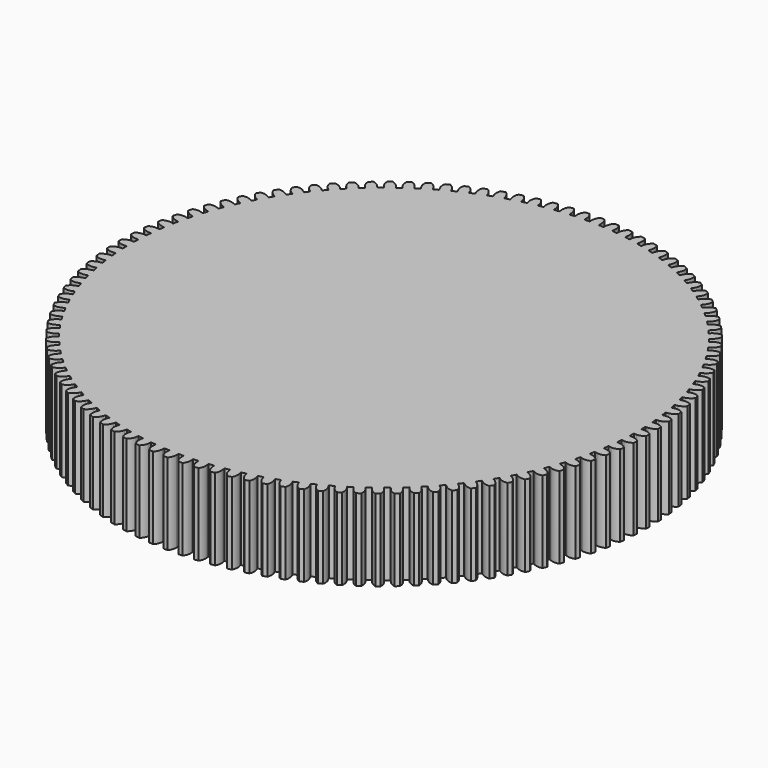
from build123d import *

# Parameters (mm, degrees)
F0_R            = 82.1730673952
F1_DEPTH        = 25.4
F3_DEPTH        = 25.4
F3_COPIES_COUNT = 110


# Not quite as in the source:
# - a pattern or mirror of a feature is missing from the dataset's text; its kind, count and spacing are read off the source's solid


with BuildPart() as f1:
    # F0 (on Top) → F1 (new body)
    with BuildSketch(Plane.XY):
        Circle(F0_R)
    extrude(amount=F1_DEPTH)

    # F2 (on face) → F3 (cut, through all)
    with BuildSketch(Plane.XY.offset(25.4)):
        with BuildLine():
            Line((-0.79375, 79.7918173952), (-0.79375, 78.9980673952))
            Line((-0.79375, 78.9980673952), (0.79375, 78.9980673952))
            Line((0.79375, 78.9980673952), (0.79375, 79.7918173952))
            ThreePointArc((0.79375, 79.7918173952), (1.0268322874, 81.0567714657), (1.6954639006, 82.155574414))
            ThreePointArc((1.6954639006, 82.155574414), (0, 82.1730673952), (-1.6954639006, 82.155574414))
            ThreePointArc((-1.6954639006, 82.155574414), (-1.0268322874, 81.0567714657), (-0.79375, 79.7918173952))
        make_face()
    f3 = extrude(amount=-F3_DEPTH, mode=Mode.SUBTRACT)

    # F3_copies: F3 ×110 about axis
    f3_copies_axis = Axis((0, 0, 0), (0, 0, 1))
    for i in range(1, F3_COPIES_COUNT):
        add(f3.rotate(f3_copies_axis, i * 360 / F3_COPIES_COUNT), mode=Mode.SUBTRACT)


solid = f1.part
